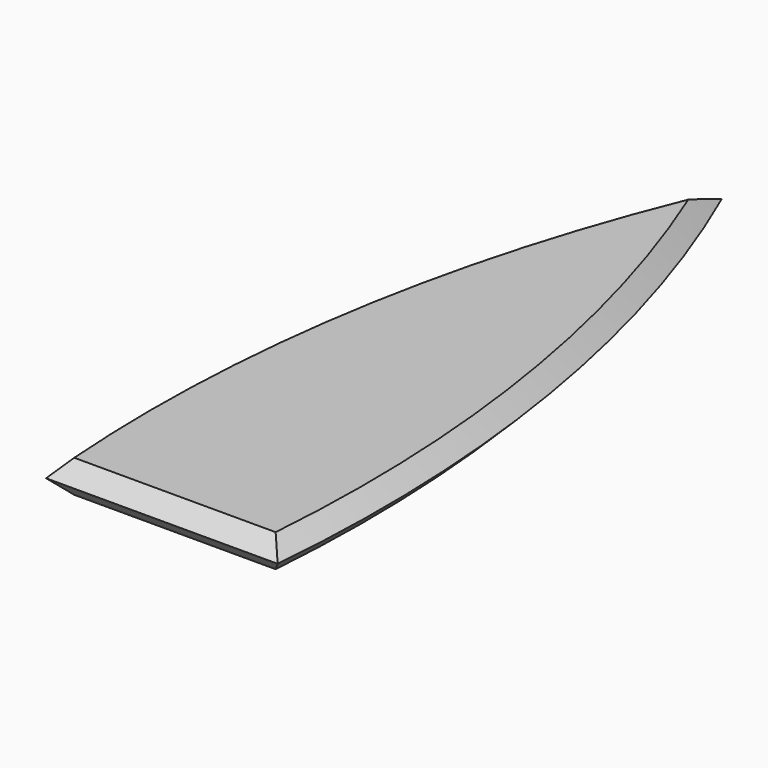
from build123d import *

# Parameters (mm, degrees)
F1_DEPTH = 3.175
F2_SIZE  = 3.17499


# Not quite as in the source:
# - a fillet or chamfer is up to 0.001 mm smaller than in the source, because OpenCascade refuses the exact size


with BuildPart() as f1:
    # F0 (on Top) → F1 (new body, symmetric)
    with BuildSketch(Plane.XY):
        with BuildLine():
            ThreePointArc((22.3162673387, -60.1211733557), (19.6694953196, 9.2531133838), (0, 75.8332006216))
            ThreePointArc((0, 75.8332006216), (-19.8842446441, 9.2801862209), (-22.7369976658, -60.1211733557))
            Line((-22.7369976658, -60.1211733557), (22.3162673387, -60.1211733557))
        make_face()
    extrude(amount=F1_DEPTH, both=True)

    # F2 (size 3.175 in the source; OpenCascade refuses exactly that, so slightly less here)
    f2_edges = [f1.edges().sort_by_distance(p)[0] for p in [
        (-0.210365, -60.121173, 3.175),
        (19.669495, 9.253113, 3.175),
        (-19.884245, 9.280186, 3.175),
        (-0.210365, -60.121173, -3.175),
        (19.669495, 9.253113, -3.175),
        (-19.884245, 9.280186, -3.175),
    ]]
    chamfer(f2_edges, length=F2_SIZE)


solid = f1.part
